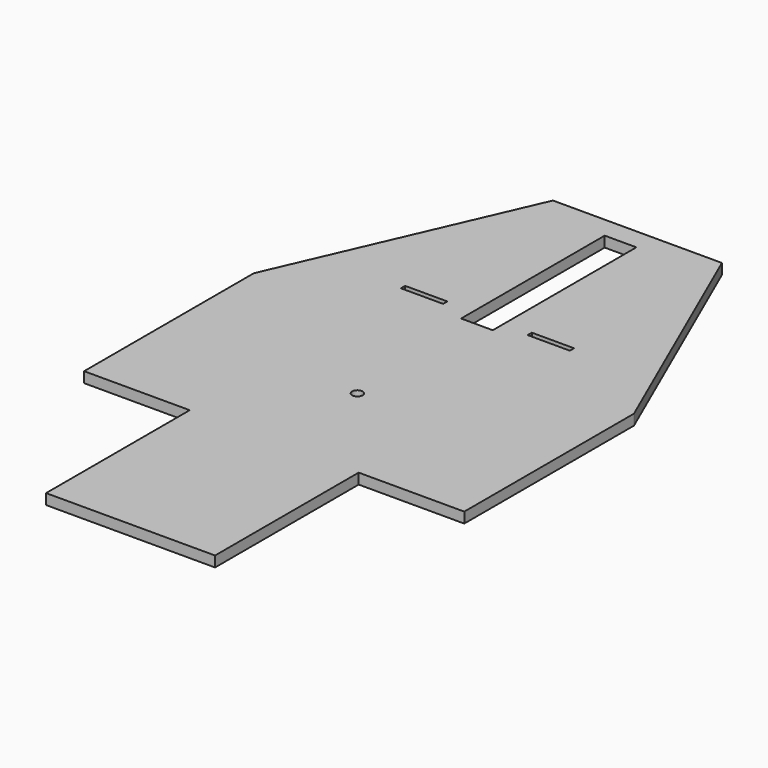
from build123d import *

# Parameters (mm, degrees)
F0_R     = 12.7
F0_W     = 50.8
F0_H     = 12.7
F0_W_2   = 63.5
F1_DEPTH = 25.4


# Not quite as in the source:
# - a feature names something its author has since deleted; it is built from what else it names


with BuildPart() as f1:
    # F0 (on Top) → F1 (new body)
    with BuildSketch(Plane.XY):
        Polygon((-406.4, -964.5238018036), (-406.4, -1396.3238018036), (0, -1396.3238018036), (0, -964.5238018036), (254, -964.5238018036), (254, -454.310915063), (0, 127.6761981964), (-406.4, 127.6761981964), (-660.4, -454.310915063), (-660.4, -964.5238018036), align=None)
        with Locations((-203.2, -714.3330844099)):
            Circle(F0_R, mode=Mode.SUBTRACT)
        Polygon((-241.3, -316.8238018036), (-241.3, 76.8761981964), (-165.1, 76.8761981964), (-165.1, -316.8238018036), (-101.6, -316.8238018036), (0, -316.8238018036), (50.8, -316.8238018036), (50.8, -329.5238018036), (0, -329.5238018036), (-101.6, -329.5238018036), (-165.1, -329.5238018036), (-165.1, -354.9238018036), (-241.3, -354.9238018036), (-241.3, -329.5238018036), (-304.8, -329.5238018036), (-406.4, -329.5238018036), (-457.2, -329.5238018036), (-457.2, -316.8238018036), (-406.4, -316.8238018036), (-304.8, -316.8238018036), align=None, mode=Mode.SUBTRACT)
        with Locations((-431.8, -323.1738018036)):
            Rectangle(F0_W, F0_H)
        with Locations((-133.35, -323.1738018036)):
            Rectangle(F0_W_2, F0_H)
        with Locations((25.4, -323.1738018036)):
            Rectangle(F0_W, F0_H)
        with Locations((-273.05, -323.1738018036)):
            Rectangle(F0_W_2, F0_H)
    extrude(amount=F1_DEPTH)


solid = f1.part
